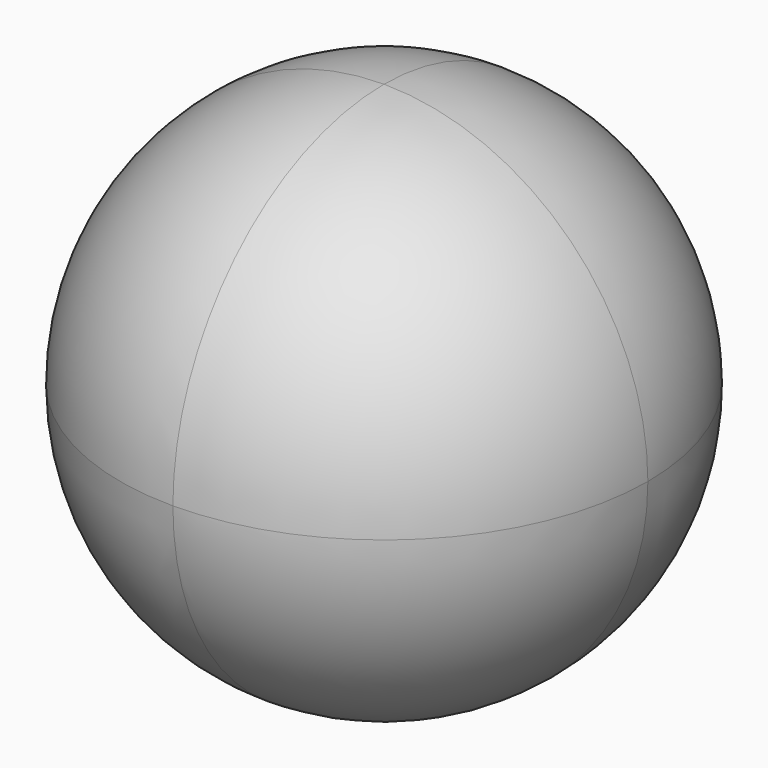
from build123d import *

# Parameters (mm, degrees)
F0_W     = 88.9
F0_H     = 88.9
F1_DEPTH = 88.9
F2_R     = 44.44999


# Not quite as in the source:
# - a fillet or chamfer is up to 0.001 mm smaller than in the source, because OpenCascade refuses the exact size


with BuildPart() as f1:
    # F0 (on Top) → F1 (new body)
    with BuildSketch(Plane.XY):
        with Locations((-67.8786515405, -18.0250238627)):
            Rectangle(F0_W, F0_H)
    extrude(amount=F1_DEPTH)

    # F2 (radius 44.45 in the source; OpenCascade refuses exactly that, so slightly less here)
    f2_edges = [f1.edges().sort_by_distance(p)[0] for p in [
        (-112.328652, -62.475024, 44.45),
        (-112.328652, 26.424976, 44.45),
        (-112.328652, -18.025024, 88.9),
        (-112.328652, -18.025024, 0),
        (-67.878652, -62.475024, 88.9),
        (-67.878652, 26.424976, 88.9),
        (-23.428652, -18.025024, 88.9),
        (-23.428652, -18.025024, 0),
        (-23.428652, 26.424976, 44.45),
        (-23.428652, -62.475024, 44.45),
        (-67.878652, -62.475024, 0),
        (-67.878652, 26.424976, 0),
    ]]
    fillet(f2_edges, radius=F2_R)


solid = f1.part
